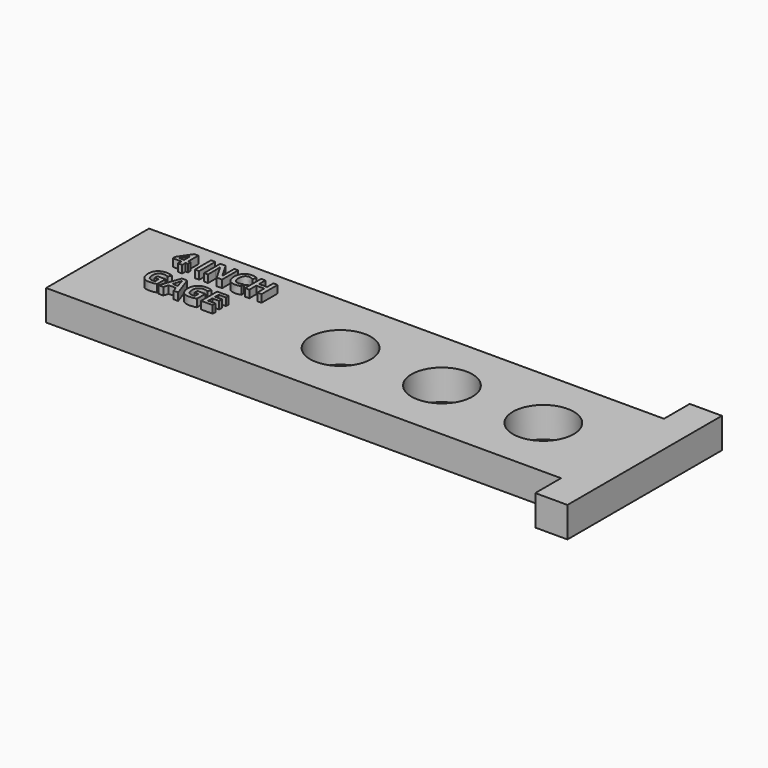
from build123d import *

# Parameters (mm, degrees)
F1_DEPTH     = 6
F2_TEXT_SIZE = 5.5555555556
F3_DEPTH     = 1.5
F5_D         = 12


# Not quite as in the source:
# - Text() gives the source's letters only with a copy of the font that has no kerning and outlines rounded to 1/6400 em; it was checked with that copy


with BuildPart() as f1:
    # F0 (on Top) → F1 (new body)
    with BuildSketch(Plane.XY):
        Polygon((-101.6, 0), (0, 0), (0, -6.35), (6.35, -6.35), (6.35, 31.75), (0, 31.75), (0, 25.4), (-101.6, 25.4), align=None)
    extrude(amount=F1_DEPTH)

    # F2 (on face) → F3 (join)
    with BuildSketch(Plane.XY.offset(6)):
        with Locations((-90.8451091361, 16.8701356886)):
            Text('4 INCH', F2_TEXT_SIZE, font='Open Sans', font_style=FontStyle.BOLD, text_align=(TextAlign.LEFT, TextAlign.BOTTOM))
        with Locations((-90.8451091361, 9.314580133)):
            Text('GAGE', F2_TEXT_SIZE, font='Open Sans', font_style=FontStyle.BOLD, text_align=(TextAlign.LEFT, TextAlign.BOTTOM))
    extrude(amount=F3_DEPTH)

    # F5 (through all)
    with Locations(Plane.XY.offset(6)):
        with Locations((-53.65, 12.7), (-33.65, 12.7), (-13.65, 12.7)):
            Hole(F5_D / 2)


solid = f1.part
